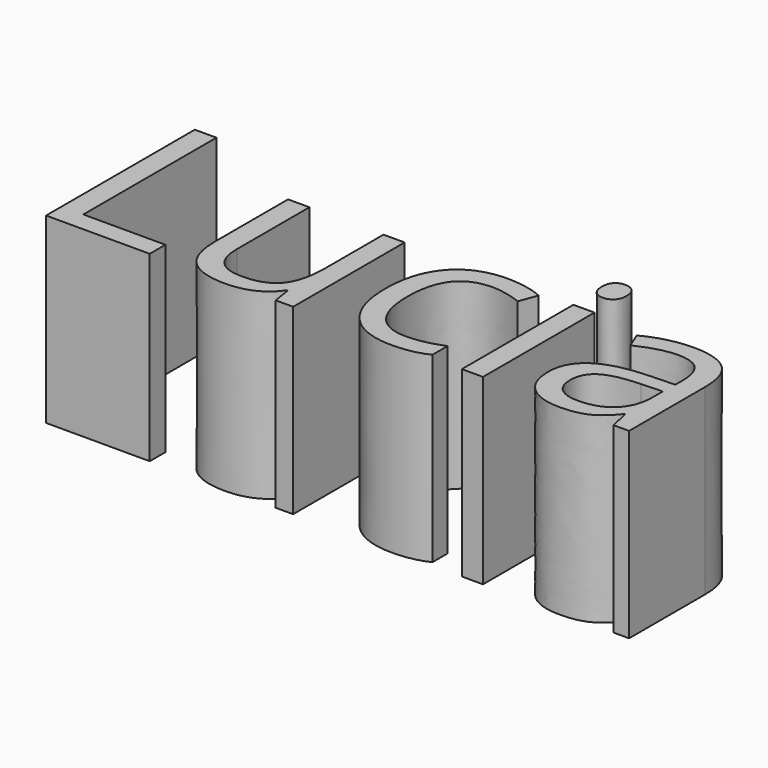
from build123d import *

# Parameters (mm, degrees)
F0_TEXT_SIZE = 13.2024909059
F1_DEPTH     = 9.2587200925


# Not quite as in the source:
# - Text() gives the source's letters only with a copy of the font that has no kerning and outlines rounded to 1/6400 em; it was checked with that copy


with BuildPart() as f1:
    # F0 (on Top) → F1 (new body)
    with BuildSketch(Plane.XY):
        with Locations((-54.6156130731, -37.7606600523)):
            Text('Lucia', F0_TEXT_SIZE, font='Open Sans', text_align=(TextAlign.LEFT, TextAlign.BOTTOM))
    extrude(amount=F1_DEPTH)


solid = f1.part
